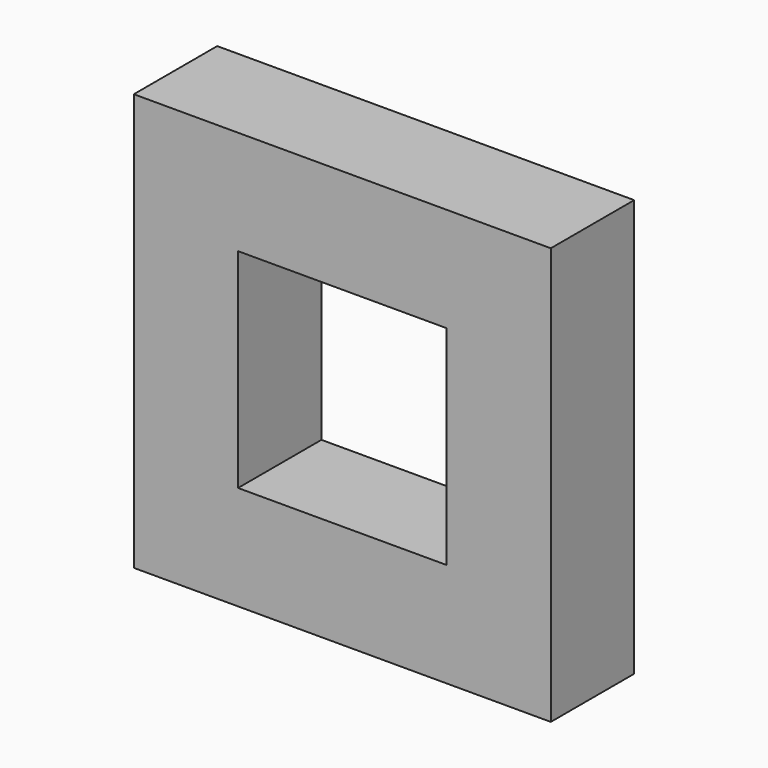
from build123d import *

# Parameters (mm, degrees)
F0_W     = 50.8
F0_H     = 50.8
F0_W_2   = 25.4
F0_H_2   = 25.4
F1_DEPTH = 12.7


# Not quite as in the source:
# - a feature names something its author has since deleted; it is built from what else it names


with BuildPart() as f1:
    # F0 (on Front) → F1 (new body)
    with BuildSketch(Plane.XZ):
        Rectangle(F0_W, F0_H)
        Rectangle(F0_W_2, F0_H_2, mode=Mode.SUBTRACT)
    extrude(amount=F1_DEPTH)


solid = f1.part
